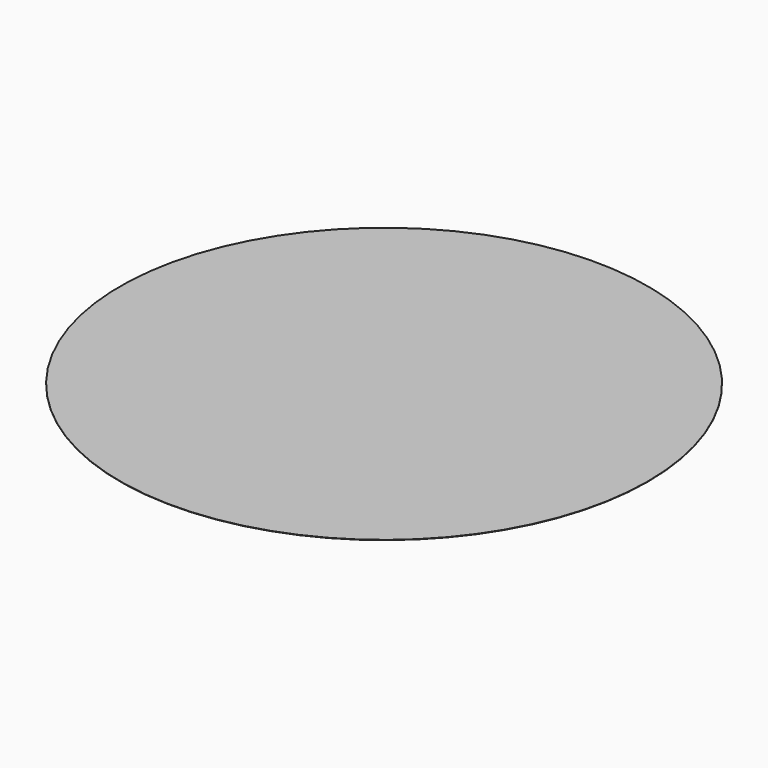
from build123d import *

# Parameters (mm, degrees)
F0_R     = 3048
F1_DEPTH = 3.175


# Not quite as in the source:
# - a length typed as a fraction of an inch, garbled in the dataset ("3 / 203.2 mm" for 3/8 in), is restored


with BuildPart() as f1:
    # F0 (on Top) → F1 (new body)
    with BuildSketch(Plane.XY):
        Circle(F0_R)
    extrude(amount=F1_DEPTH)


solid = f1.part
